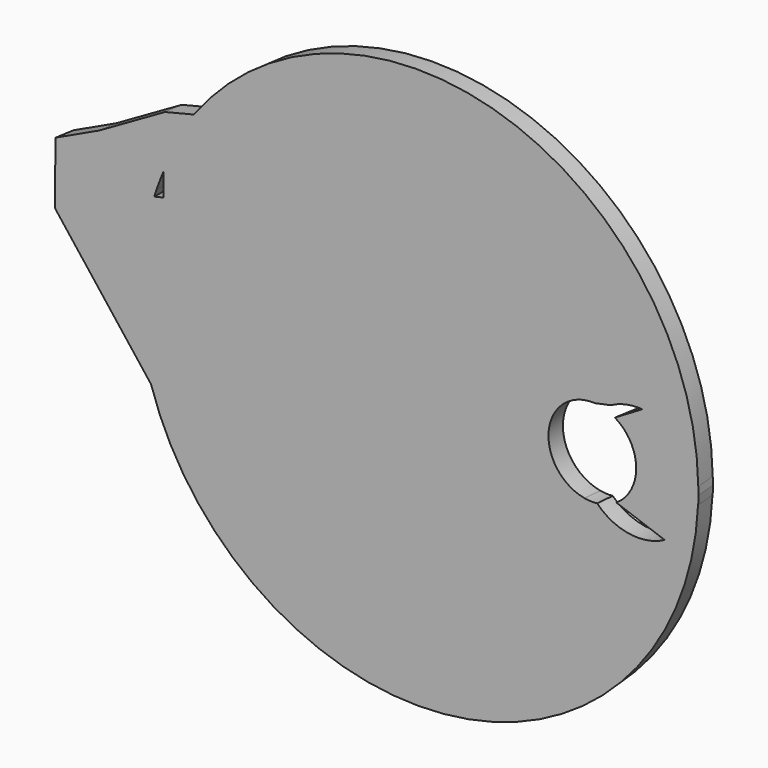
from build123d import *

# Parameters (mm, degrees)
F1_DEPTH               = 12.7
DRAFT_F1_DRAFTED_ANGLE = -5


# Not quite as in the source:
# - an extrude with a draft is written as a straight extrude whose walls are then drafted


with BuildPart() as f1:
    # F0 (on Front) → F1 (new body)
    with BuildSketch(Plane.XZ):
        with BuildLine():
            Line((108.3981027489, 28.5980702669), (0, 174.3752223149))
            ThreePointArc((0, 174.3752223149), (-78.3368206298, 155.7885127055), (-139.973748724, 103.9907102848))
            ThreePointArc((-139.973748724, 103.9907102848), (-150.0148868924, 88.894611018), (-158.4342652368, 72.8375024027))
            Line((-158.4342652368, 72.8375024027), (-158.5001747821, 52.0825752072))
            Line((-158.5001747821, 52.0825752072), (-167.0124556551, 50.1353948169))
            ThreePointArc((-167.0124556551, 50.1353948169), (-174.3726257545, -0.951601216), (-166.4553179949, -51.9552236893))
            ThreePointArc((-166.4553179949, -51.9552236893), (-103.312667365, -140.4749476573), (0, -174.3752223149))
            Line((0, -174.3752223149), (126.8824701646, -61.2326356398))
            Line((126.8824701646, -61.2326356398), (103.89653358, -28.1330077059))
            ThreePointArc((103.89653358, -28.1330077059), (80.7668968438, -4.0993384936), (96.1294818343, 25.5078959899))
            ThreePointArc((96.1294818343, 25.5078959899), (102.0908123385, 27.739748754), (108.3981027489, 28.5980702669))
        make_face()
        with BuildLine():
            ThreePointArc((174.3567412746, 2.5386865644), (122.401050084, 124.1962201346), (0, 174.3752223149))
            Line((0, 174.3752223149), (108.3981027489, 28.5980702669))
            ThreePointArc((108.3981027489, 28.5980702669), (109.4561605031, 28.603643945), (110.5137006242, 28.5700854961))
            Line((110.5137006242, 28.5700854961), (120.1951823061, 30.6311311493))
            ThreePointArc((120.1951823061, 30.6311311493), (125.6991471994, 33.0137654184), (131.515544177, 34.4766740982))
            ThreePointArc((131.515544177, 34.4766740982), (137.6103873734, 34.9816749113), (143.7052305697, 34.4766740982))
            ThreePointArc((143.7052305697, 34.4766740982), (164.3283739015, 23.5916870861), (174.3567412746, 2.5386865644))
        make_face()
        with BuildLine():
            ThreePointArc((-158.4342652368, 72.8375024027), (-150.0148868924, 88.894611018), (-139.973748724, 103.9907102848))
            Line((-139.973748724, 103.9907102848), (-158.3498808299, 99.4101666848))
            Line((-158.3498808299, 99.4101666848), (-158.4342652368, 72.8375024027))
        make_face()
        with BuildLine():
            ThreePointArc((174.6421489395, -2.0500866548), (174.570728151, 0.2487335422), (174.3567412746, 2.5386865644))
            ThreePointArc((174.3567412746, 2.5386865644), (174.3706019936, 1.2693769162), (174.3752223149, 0))
            ThreePointArc((174.3752223149, 0), (174.3323462466, -3.8666793928), (174.2037391268, -7.7314572768))
            ThreePointArc((174.2037391268, -7.7314572768), (174.53238381, -4.8992170181), (174.6421489395, -2.0500866548))
        make_face()
        with BuildLine():
            ThreePointArc((174.3752223149, 0), (174.3706019936, 1.2693769162), (174.3567412746, 2.5386865644))
            ThreePointArc((174.3567412746, 2.5386865644), (164.3283739015, 23.5916870861), (143.7052305697, 34.4766740982))
            Line((143.7052305697, 34.4766740982), (125.3227635033, 23.5459688319))
            ThreePointArc((125.3227635033, 23.5459688319), (134.4058194937, 13.2967232616), (137.6839426441, 0))
            ThreePointArc((137.6839426441, 0), (134.7462483555, -12.627041518), (126.5365356636, -22.6606272553))
            Line((126.5365356636, -22.6606272552), (157.0932145337, -33.5424795544))
            ThreePointArc((157.0932145337, -33.5424795544), (168.4760102918, -22.511383939), (174.2037391268, -7.7314572768))
            ThreePointArc((174.2037391268, -7.7314572768), (174.3323462466, -3.8666793928), (174.3752223149, 0))
        make_face()
        with BuildLine():
            ThreePointArc((-165.1545177599, 55.9526891299), (-162.0145035179, 64.4827016125), (-158.4342652368, 72.8375024027))
            Line((-158.4342652368, 72.8375024027), (-158.3498808299, 99.4101666848))
            Line((-158.3498808299, 99.4101666848), (-199.4119243255, 75.8765293267))
            Line((-199.4119243255, 75.8765293267), (-165.1545177599, 55.9526891299))
        make_face()
        with BuildLine():
            ThreePointArc((-167.0124556551, 50.1353948169), (-166.1089545605, 53.052175942), (-165.1545177599, 55.9526891299))
            Line((-165.1545177599, 55.9526891299), (-199.4119243255, 75.8765293267))
            Line((-199.4119243255, 75.8765293267), (-226.1803895235, 63.3067376912))
            Line((-226.1803895235, 63.3067376912), (-193.6574989016, 44.0403532548))
            Line((-193.6574989016, 44.0403532548), (-167.0124556551, 50.1353948169))
        make_face()
        with BuildLine():
            ThreePointArc((0, -174.3752223149), (120.5374289918, -126.0057394305), (174.2037391268, -7.7314572768))
            ThreePointArc((174.2037391268, -7.7314572768), (168.4760102918, -22.511383939), (157.0932145337, -33.5424795544))
            ThreePointArc((157.0932145337, -33.5424795544), (133.5137679356, -38.8545574957), (111.6795194331, -28.4875875307))
            ThreePointArc((111.6795194331, -28.4875875307), (107.775898519, -28.5765055322), (103.89653358, -28.1330077059))
            Line((103.89653358, -28.1330077059), (126.8824701646, -61.2326356398))
            Line((126.8824701646, -61.2326356398), (0, -174.3752223149))
        make_face()
        with BuildLine():
            ThreePointArc((-166.4553179949, -51.9552236893), (-174.3726257545, -0.951601216), (-167.0124556551, 50.1353948169))
            Line((-167.0124556551, 50.1353948169), (-193.6574989016, 44.0403532548))
            Line((-193.6574989016, 44.0403532548), (-226.6041225736, 25.5078959899))
            Line((-226.6041225736, 25.5078959899), (-166.4553179949, -51.9552236893))
        make_face()
        Polygon((-193.6574989016, 44.0403532548), (-226.1803895235, 63.3067376912), (-226.6041225736, 25.5078959899), align=None)
    extrude(amount=F1_DEPTH)

    # draft_F1_drafted
    draft_f1_drafted_walls = [f1.faces().sort_by_distance(p)[0] for p in [
        (-196.5297202842, -8.4666666667, -13.2236638497),
        (22.4487168104, -8.4666666667, -172.924183592),
        (174.6380401481, -8.4666666667, -2.6017157743),
        (53.5600207564, -8.4666666667, 165.9459018294),
        (-149.1618147769, -8.4666666667, 101.7004384848),
        (-178.8809025777, -8.4666666667, 87.6433480058),
        (-212.7961569245, -8.4666666667, 69.5916335089),
        (-226.3922560485, -8.4666666667, 44.4073168405),
        (141.8148750986, -8.4666666667, -28.1015534048),
        (133.5137679356, -8.4666666667, -38.8545574957),
        (80.4776193909, -8.4666666667, -0.5843670528),
        (115.3544414652, -8.4666666667, 29.6006083227),
        (131.6325367258, -8.4666666667, 34.4960029627),
        (134.5139970365, -8.4666666667, 29.011321465),
        (137.6740782352, -8.4666666667, 0.7511778358),
        (-162.7563152186, -8.4666666667, 51.1089850121),
        (-163.11878634, -8.4666666667, 61.6358637512),
        (-158.4672200095, -8.4666666667, 62.460038805),
    ]]
    draft(draft_f1_drafted_walls, neutral_plane=Plane.XZ, angle=DRAFT_F1_DRAFTED_ANGLE)


solid = f1.part
